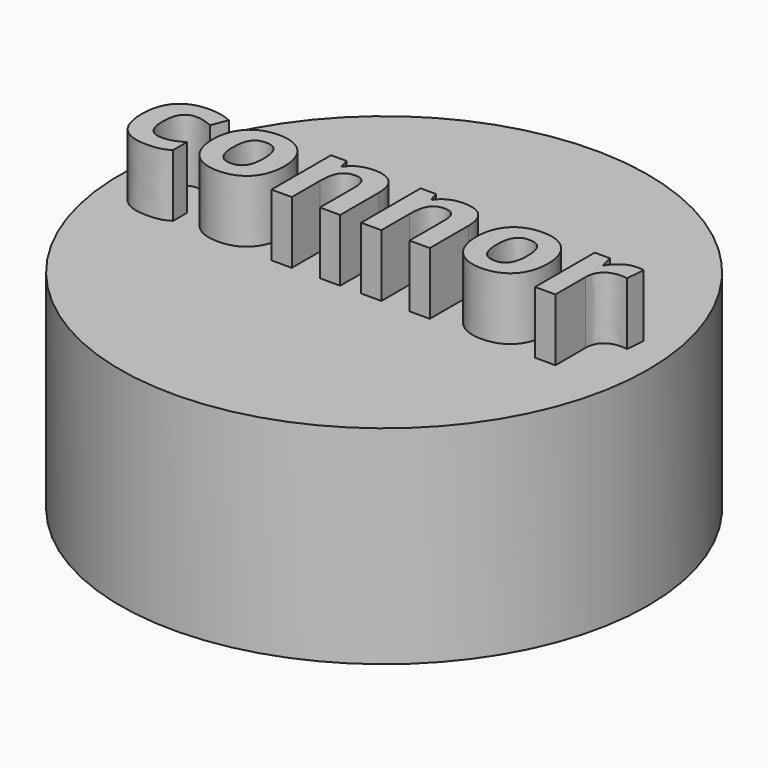
from build123d import *

# Parameters (mm, degrees)
F0_R         = 25.4201285058
F1_DEPTH     = 20
F2_TEXT_SIZE = 13.1302526117
F3_DEPTH     = 6


# Not quite as in the source:
# - Text() gives the source's letters only with a copy of the font that has no kerning and outlines rounded to 1/6400 em; it was checked with that copy


with BuildPart() as f1:
    # F0 (on Top) → F1 (new body)
    with BuildSketch(Plane.XY):
        Circle(F0_R)
    extrude(amount=F1_DEPTH)

    # F2 (on face) → F3 (join)
    with BuildSketch(Plane.XY.offset(20)):
        with Locations((-23.7289946526, -3.7815128453)):
            Text('connor', F2_TEXT_SIZE, font='Open Sans', font_style=FontStyle.BOLD, text_align=(TextAlign.LEFT, TextAlign.BOTTOM))
    extrude(amount=F3_DEPTH)


solid = f1.part
